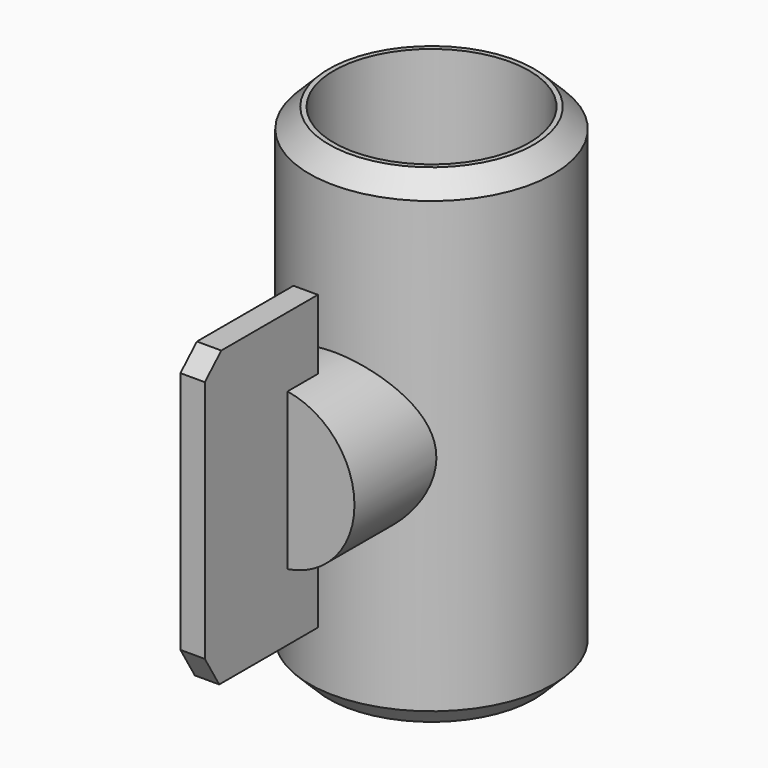
from build123d import *

# Parameters (mm, degrees)
F0_R     = 12.5
F1_DEPTH = 50
F2_SIZE  = 2
F3_R     = 8.1072881944
F4_DEPTH = 20
F5_R     = 10
F6_DEPTH = 50.001
F8_DEPTH = 1.25


with BuildPart() as f1:
    # F0 (on Top) → F1 (new body)
    with BuildSketch(Plane.XY):
        Circle(F0_R)
    extrude(amount=F1_DEPTH)

    # F2
    f2_edges = [f1.edges().sort_by_distance(p)[0] for p in [
        (-12.5, 0, 50),
        (-12.5, 0, 0),
    ]]
    chamfer(f2_edges, length=F2_SIZE)

    # F3 (on Front) → F4 (join)
    with BuildSketch(Plane.XZ):
        with Locations((0, 24.8591881245)):
            Circle(F3_R)
    extrude(amount=F4_DEPTH)

    # F5 (on face) → F6 (cut, through all)
    with BuildSketch(Plane.XY.offset(50)):
        Circle(F5_R)
    extrude(amount=-F6_DEPTH, mode=Mode.SUBTRACT)

    # F7 (on Right) → F8 (join, symmetric)
    with BuildSketch(Plane.YZ):
        Polygon((-16.112501399, 40), (-28.4739788622, 40), (-30.5820492643, 38.0051359534), (-30.5820492643, 13.057355769), (-28.7352129817, 10), (-16.112501399, 10), align=None)
    extrude(amount=F8_DEPTH, both=True)


solid = f1.part
